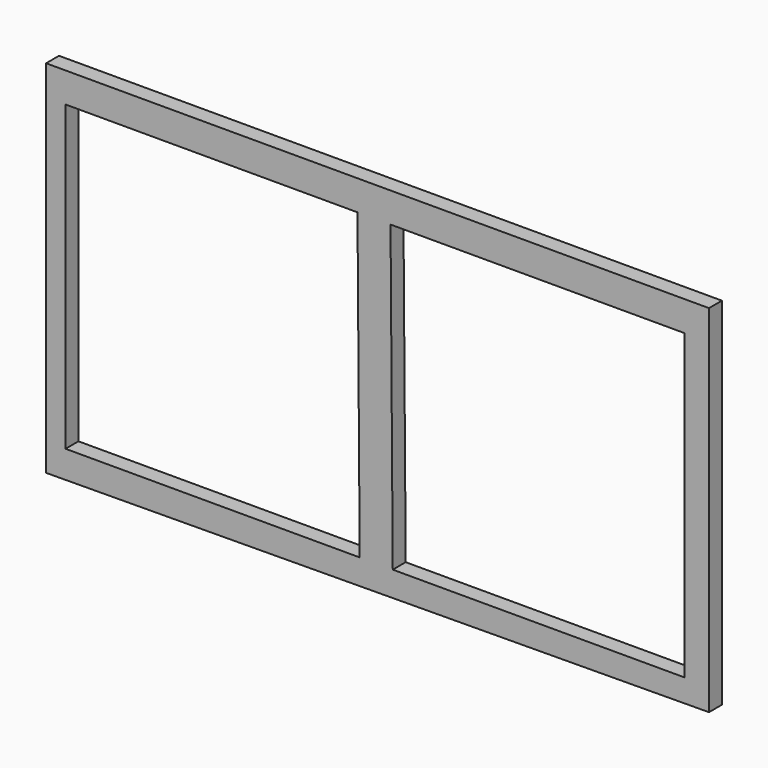
from build123d import *

# Parameters (mm, degrees)
F1_DEPTH = 2.54


# Not quite as in the source:
# - a feature names something its author has since deleted; it is built from what else it names


with BuildPart() as f1:
    # F0 (on Front) → F1 (new body)
    with BuildSketch(Plane.XZ):
        Polygon((-45.7926876843, 0), (-48.8455332816, 0), (-48.8455332816, -56.6048510373), (-45.7926876843, -56.5824585276), (-45.7926876843, -52.2799864411), (-45.7926876843, -32.4403391187), (-45.7926876843, -28.3024255186), (-45.7926876843, -4.7043516129), align=None)
        Polygon((0, 0), (-45.7926876843, 0), (-45.7926876843, -4.7043516129), (0.0345062453, -4.7043516129), align=None)
        Polygon((-45.7926876843, -52.2799864411), (-45.7926876843, -56.5824585276), (5.5995524852, -56.2054983442), (5.5707590003, -52.2799864411), (0.3834717695, -52.2799864411), align=None)
        Polygon((5.1872872309, 0), (0, 0), (0.0345062453, -4.7043516129), (5.2217934762, -4.7043516129), align=None)
        Polygon((5.5707590003, -52.2799864411), (5.5995524852, -56.2054983442), (51.3895750046, -55.8696302204), (51.3895750046, -52.2799864411), align=None)
        Polygon((51.3895750046, 0), (5.1872872309, 0), (5.2217934762, -4.7043516129), (51.3895750046, -4.7043516129), align=None)
        Polygon((51.3895750046, -52.2799864411), (51.3895750046, -55.8696302204), (55.2056245506, -55.8416396379), (55.2056245506, 0), (51.3895750046, 0), (51.3895750046, -4.7043516129), (51.3895750046, -28.3024255186), align=None)
        Polygon((5.2217934762, -4.7043516129), (0.0345062453, -4.7043516129), (0.2379486892, -32.4403391187), (0.3834717695, -52.2799864411), (5.5707590003, -52.2799864411), align=None)
    extrude(amount=F1_DEPTH)


solid = f1.part
